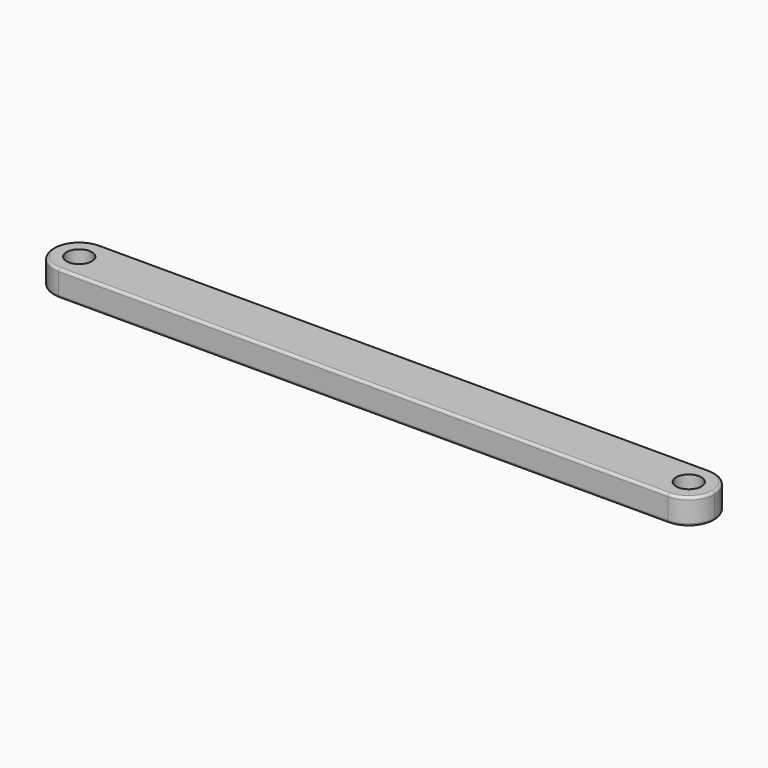
from build123d import *

# Parameters (mm, degrees)
F0_W     = 51
F0_H     = 4
F1_DEPTH = 2
F2_R     = 1.99999
F3_R     = 0.969
F4_DEPTH = 25
F5_R     = 0.2


# Not quite as in the source:
# - a fillet or chamfer is up to 0.001 mm smaller than in the source, because OpenCascade refuses the exact size


with BuildPart() as f1:
    # F0 (on Top) → F1 (new body)
    with BuildSketch(Plane.XY):
        with Locations((2.7281418443, -3.9396004599)):
            Rectangle(F0_W, F0_H)
    extrude(amount=F1_DEPTH)

    # F2 (radius 2 in the source; OpenCascade refuses exactly that, so slightly less here)
    f2_edges = [f1.edges().sort_by_distance(p)[0] for p in [
        (28.228142, -1.9396, 1),
        (28.228142, -5.9396, 1),
        (-22.771858, -1.9396, 1),
        (-22.771858, -5.9396, 1),
    ]]
    fillet(f2_edges, radius=F2_R)

    # F3 (on face) → F4 (cut)
    with BuildSketch(Plane.XY.offset(2)):
        with Locations((-20.7718581557, -3.9396004599)):
            Circle(F3_R)
        with Locations((26.2281418443, -3.9396004599)):
            Circle(F3_R)
    extrude(amount=-F4_DEPTH, mode=Mode.SUBTRACT)

    # F5
    f5_edges = [f1.edges().sort_by_distance(p)[0] for p in [
        (2.728142, -1.9396, 0),
        (2.728142, -5.9396, 2),
    ]]
    fillet(f5_edges, radius=F5_R)


solid = f1.part
